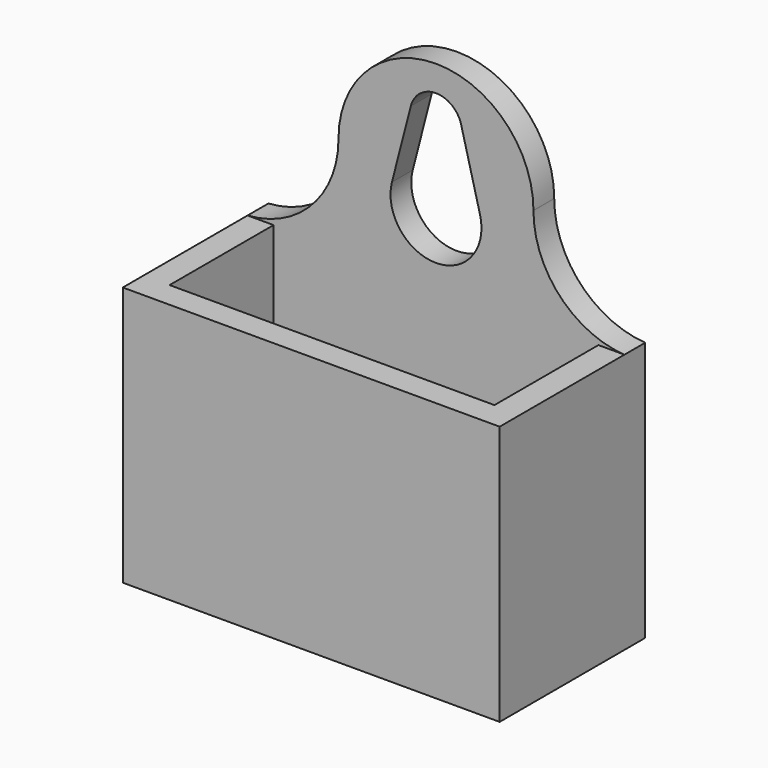
from build123d import *

# Parameters (mm, degrees)
F0_W        = 29
F0_H        = 14
F0_W_2      = 25
F0_H_2      = 10
F1_DEPTH    = 20
F2_W        = 15
F2_H        = 2
F3_DEPTH    = 15
F5_DEPTH    = 2
F6_T1_DEPTH = 2
F6_T3_DEPTH = 2
F6_T5_DEPTH = 39.5
F6_T7_DEPTH = 39.5


# Not quite as in the source:
# - a fillet or chamfer that OpenCascade refuses, or shapes differently, is made with other operations: its cross-section is extruded or revolved along the edge and cut away or added


with BuildPart() as f1:
    # F0 (on Top) → F1 (new body)
    with BuildSketch(Plane.XY):
        with Locations((14.5, -7)):
            Rectangle(F0_W, F0_H)
        with Locations((14.5, -7)):
            Rectangle(F0_W_2, F0_H_2, mode=Mode.SUBTRACT)
    extrude(amount=F1_DEPTH)

    # F2 (on face) → F3 (join)
    with BuildSketch(Plane.XY.offset(20)):
        with Locations((14.5, -1)):
            Rectangle(F2_W, F2_H)
    extrude(amount=F3_DEPTH)

    # F4 (on face) → F5 (cut, through all)
    with BuildSketch(Plane.XZ.offset(2)):
        with BuildLine():
            Line((17.8888604279, 25.875), (16.4364916731, 31.5))
            ThreePointArc((16.4364916731, 31.5), (14.5, 33), (12.5635083269, 31.5))
            Line((12.5635083269, 31.5), (11.1111395721, 25.875))
            ThreePointArc((11.1111395721, 25.875), (14.5, 21.5), (17.8888604279, 25.875))
        make_face()
    extrude(amount=-F5_DEPTH, mode=Mode.SUBTRACT)

    # F6: fillet of radius 7.5 on 4 edges, made by hand

    # F6_s2 → F6_t1 (join)
    with BuildSketch(Plane.XZ):
        with BuildLine():
            ThreePointArc((0, 20), (4.9772255751, 22.3598393906), (7, 27.4833147735))
            Line((7, 27.4833147735), (7, 20))
            Line((7, 20), (0, 20))
        make_face()
    extrude(amount=F6_T1_DEPTH)

    # F6_s4 → F6_t3 (join)
    with BuildSketch(Plane.XZ):
        with BuildLine():
            ThreePointArc((29, 20), (24.0227744249, 22.3598393906), (22, 27.4833147735))
            Line((22, 27.4833147735), (22, 20))
            Line((22, 20), (29, 20))
        make_face()
    extrude(amount=F6_T3_DEPTH)

    # F6_s6 → F6_t5 (cut)
    with BuildSketch(Plane.XZ.offset(-18.75)):
        with BuildLine():
            ThreePointArc((22, 27.5), (19.8033008589, 32.8033008589), (14.5, 35))
            Line((14.5, 35), (22, 35))
            Line((22, 35), (22, 27.5))
        make_face()
    extrude(amount=F6_T5_DEPTH, mode=Mode.SUBTRACT)

    # F6_s8 → F6_t7 (cut)
    with BuildSketch(Plane.XZ.offset(-18.75)):
        with BuildLine():
            ThreePointArc((7, 27.5), (9.1966991411, 32.8033008589), (14.5, 35))
            Line((14.5, 35), (7, 35))
            Line((7, 35), (7, 27.5))
        make_face()
    extrude(amount=F6_T7_DEPTH, mode=Mode.SUBTRACT)


solid = f1.part
